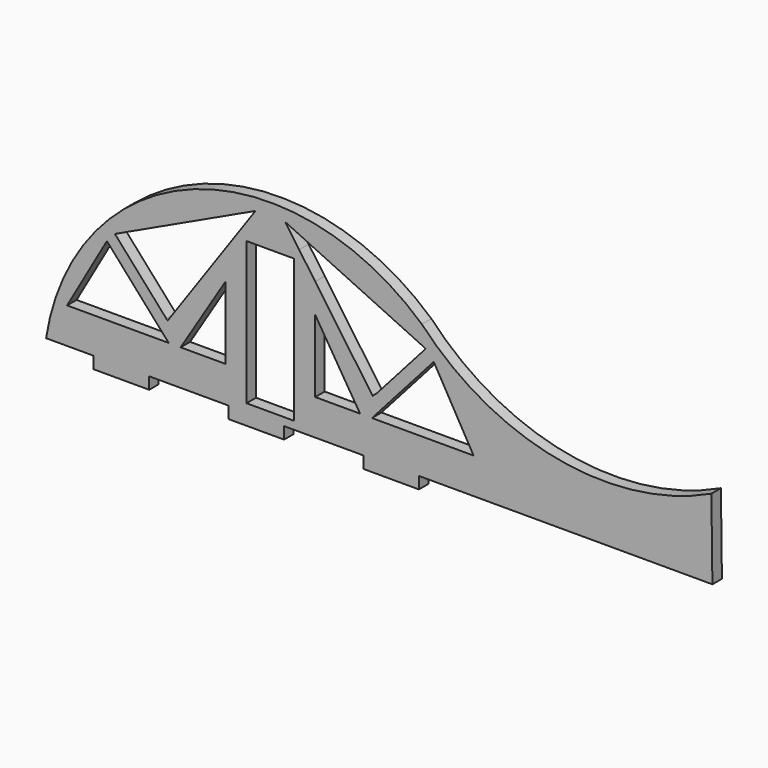
from build123d import *

# Parameters (mm, degrees)
F1_DEPTH = 19.05
F3_DEPTH = 25.4
F4_W     = 88.9
F4_H     = 19.05
F4_W_2   = 38.1
F4_H_2   = 44.45
F5_DEPTH = 19.05
F6_DEPTH = 25.4


with BuildPart() as f1:
    # F0 (on Front) → F1 (new body)
    with BuildSketch(Plane.XZ):
        with BuildLine():
            Line((754.4526390882, -127), (1219.7509574175, -127))
            Line((1219.7509574175, -127), (1218.1324014764, 0.3078377019))
            ThreePointArc((1218.1324014764, 0.3078377019), (971.9574719259, -30.9690211882), (754.4526390882, 88.4963944497))
            Line((754.4526390882, 88.4963944497), (754.4526390882, -127))
        make_face()
        with BuildLine():
            Line((152.9509574175, -127), (754.4526390882, -127))
            Line((754.4526390882, -127), (754.4526390882, 88.4963944497))
            ThreePointArc((754.4526390882, 88.4963944497), (389.4863986152, 159.9886479518), (152.9509574175, -127))
        make_face()
    extrude(amount=F1_DEPTH)

    # F2 (on face) → F3 (cut)
    with BuildSketch(Plane.XZ.offset(19.05)):
        Polygon((349.2892183732, -69.85), (250.3213995681, 41.6179700068), (186.5879998116, -69.85), (250.3213995681, -69.85), (313.393828538, -69.85), (314.0547993247, -69.85), align=None)
        Polygon((398.7721789756, 33.9153755605), (456.7740343957, 116.6469860451), (488.14527835, 161.3937189979), (263.1718880821, 55.8370334618), (275.3515595595, 42.1190060128), (321.7644516922, -10.1560762376), (345.300821131, -36.6652117763), (347.0743577182, -38.6627552758), (347.5783524621, -39.1055249546), (349.2892183732, -36.6652117763), align=None)
        Polygon((511.9904369348, 162.2207457014), (368.3392183732, -69.85), (655.6416554964, -69.85), align=None)
        Polygon((535.8355955196, 161.3937189979), (558.164750711, 129.544272866), (618.0461857734, 44.1317024412), (675.8040291483, -38.2518586693), (682.4792207708, -32.3878542947), (696.5108706698, -16.5849944314), (738.8565177121, 31.1059279369), (760.8124771809, 55.8333800289), align=None)
        Polygon((837.3928740579, -69.85), (773.6627312413, 41.6141579413), (674.6916554964, -69.85), align=None)
    extrude(amount=-F3_DEPTH, mode=Mode.SUBTRACT)

    # F4 (on face) → F5 (join)
    with BuildSketch(Plane.XZ.offset(19.05)):
        with Locations((705.4009574175, -136.525)):
            Rectangle(F4_W, F4_H)
        with Locations((489.5009574175, -136.525)):
            Rectangle(F4_W, F4_H)
        Polygon((250.3213995681, -127), (229.1509574175, -127), (229.1509574175, -146.05), (318.0509574175, -146.05), (318.0509574175, -127), align=None)
        Polygon((583.8160462156, -69.85), (655.6416554964, -69.85), (583.8160462156, 46.1853728507), align=None)
        Polygon((583.8160462156, -69.85), (583.8160462156, 46.1853728507), (550.0904369348, 100.6696116438), (550.0904369348, -69.85), align=None)
        Polygon((550.0904369348, 100.6696116438), (583.8160462156, 46.1853728507), (583.8160462156, 92.9562538667), (578.4083301084, 100.6696116438), align=None)
        Polygon((550.0904369348, -69.85), (550.0904369348, 100.6696116438), (541.6532601983, 114.3), (511.9904369348, 114.3), (511.9904369348, -69.85), align=None)
        Polygon((541.6532601983, 114.3), (550.0904369348, 100.6696116438), (550.0904369348, 114.3), align=None)
        Polygon((578.4083301084, 100.6696116438), (583.8160462156, 92.9562538667), (618.0461857734, 44.1317024412), (675.8040291483, -38.2518586693), (682.4792207708, -32.3878542947), (696.5108706698, -16.5849944314), (738.8565177121, 31.1059279369), (760.8124771809, 55.8333800289), (535.8355955196, 161.3937189979), (558.164750711, 129.544272866), align=None)
        with Locations((531.0404369348, -92.075)):
            Rectangle(F4_W_2, F4_H_2)
        Polygon((511.9904369348, 114.3), (541.6532601983, 114.3), (511.9904369348, 162.2207457014), (482.3276136712, 114.3), align=None)
        with Locations((492.9404369348, -92.075)):
            Rectangle(F4_W_2, F4_H_2)
        Polygon((473.8904369348, -69.85), (511.9904369348, -69.85), (511.9904369348, 114.3), (482.3276136712, 114.3), (473.8904369348, 100.6696116438), align=None)
        Polygon((440.164827654, -69.85), (473.8904369348, -69.85), (473.8904369348, 100.6696116438), (440.164827654, 46.1853728507), align=None)
        Polygon((473.8904369348, 100.6696116438), (482.3276136712, 114.3), (473.8904369348, 114.3), align=None)
        Polygon((368.3392183732, -69.85), (440.164827654, -69.85), (440.164827654, 46.1853728507), align=None)
        Polygon((440.164827654, 46.1853728507), (473.8904369348, 100.6696116438), (445.5725437612, 100.6696116438), (440.164827654, 92.9562538667), align=None)
    extrude(amount=-F5_DEPTH)

    # F4 (on face) → F6 (cut)
    with BuildSketch(Plane.XZ.offset(19.05)):
        Polygon((583.8160462156, -69.85), (655.6416554964, -69.85), (583.8160462156, 46.1853728507), align=None)
        Polygon((550.0904369348, -69.85), (550.0904369348, 100.6696116438), (541.6532601983, 114.3), (511.9904369348, 114.3), (511.9904369348, -69.85), align=None)
        Polygon((541.6532601983, 114.3), (550.0904369348, 100.6696116438), (550.0904369348, 114.3), align=None)
        Polygon((578.4083301084, 100.6696116438), (583.8160462156, 92.9562538667), (618.0461857734, 44.1317024412), (675.8040291483, -38.2518586693), (682.4792207708, -32.3878542947), (696.5108706698, -16.5849944314), (738.8565177121, 31.1059279369), (760.8124771809, 55.8333800289), (535.8355955196, 161.3937189979), (558.164750711, 129.544272866), align=None)
        with Locations((531.0404369348, -92.075)):
            Rectangle(F4_W_2, F4_H_2)
        with Locations((492.9404369348, -92.075)):
            Rectangle(F4_W_2, F4_H_2)
        Polygon((473.8904369348, -69.85), (511.9904369348, -69.85), (511.9904369348, 114.3), (482.3276136712, 114.3), (473.8904369348, 100.6696116438), align=None)
        Polygon((473.8904369348, 100.6696116438), (482.3276136712, 114.3), (473.8904369348, 114.3), align=None)
        Polygon((368.3392183732, -69.85), (440.164827654, -69.85), (440.164827654, 46.1853728507), align=None)
    extrude(amount=-F6_DEPTH, mode=Mode.SUBTRACT)


solid = f1.part
